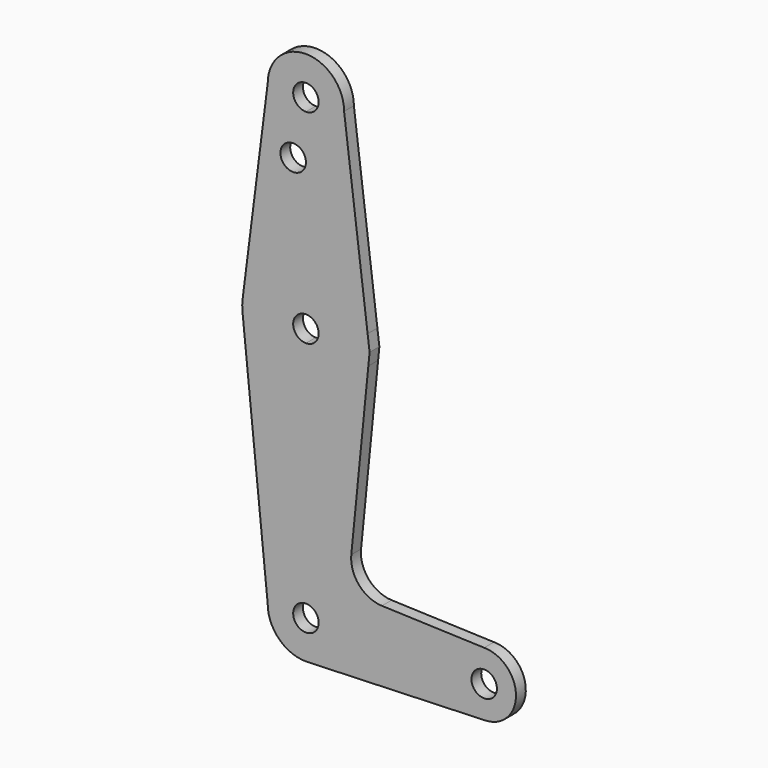
from build123d import *

# Parameters (mm, degrees)
F0_R     = 3.175
F1_DEPTH = 3.048


with BuildPart() as f1:
    # F0 (on Front) → F1 (new body)
    with BuildSketch(Plane.XZ):
        with BuildLine():
            ThreePointArc((0, 3.175), (2.2450640303, 2.2450640303), (3.175, 0))
            Line((3.175, 0), (9.525, 0))
            ThreePointArc((9.525, 0), (6.7351920908, 6.7351920908), (0, 9.525))
            Line((0, 9.525), (0, 3.175))
        make_face()
        with BuildLine():
            Line((9.525, 0), (3.175, 0))
            ThreePointArc((3.175, 0), (-2.2450640303, -2.2450640303), (0, 3.175))
            Line((0, 3.175), (0, 9.525))
            ThreePointArc((0, 9.525), (-6.7351920908, 6.7351920908), (-9.525, 0))
            ThreePointArc((-9.525, 0), (-6.7351920908, -6.7351920908), (0, -9.525))
            Line((0, -9.525), (0.6773435479, -9.500885786))
            ThreePointArc((0.6773435479, -9.500885786), (6.9705567315, -6.4912990883), (9.525, 0))
        make_face()
        with BuildLine():
            ThreePointArc((0, 9.525), (6.7351920908, 6.7351920908), (9.525, 0))
            Line((9.525, 0), (36.5125, 0))
            ThreePointArc((36.5125, 0), (38.8373399243, 5.6126600757), (44.45, 7.9375))
            Line((44.45, 7.9375), (18.9443021901, 8.8484177789))
            ThreePointArc((18.9443021901, 8.8484177789), (13.2409930554, 11.562802358), (11.3167370079, 17.5788523406))
            Line((11.3167370079, 17.5788523406), (15.5652161214, 60.3791552277))
            ThreePointArc((15.5652161214, 60.3791552277), (10.0616155323, 51.22076884), (0, 47.625))
            Line((0, 47.625), (0, 9.525))
        make_face()
        with BuildLine():
            Line((36.5125, 0), (9.525, 0))
            ThreePointArc((9.525, 0), (6.9705567315, -6.4912990883), (0.6773435479, -9.500885786))
            Line((0.6773435479, -9.500885786), (44.7324052746, -7.9324746146))
            ThreePointArc((44.7324052746, -7.9324746146), (38.9380895153, -5.7116327839), (36.5125, 0))
        make_face()
        with BuildLine():
            ThreePointArc((-9.525, 0), (-6.7351920908, 6.7351920908), (0, 9.525))
            Line((0, 9.525), (0, 47.625))
            ThreePointArc((0, 47.625), (-10.6447561055, 51.7227001204), (-15.7942028094, 61.9003804782))
            Line((-15.7942028094, 61.9003804782), (-9.525, 0))
        make_face()
        with BuildLine():
            ThreePointArc((44.45, 7.9375), (38.8373399243, 5.6126600757), (36.5125, 0))
            ThreePointArc((36.5125, 0), (38.9380895153, -5.7116327839), (44.7324052746, -7.9324746146))
            ThreePointArc((44.7324052746, -7.9324746146), (50.1616327839, -5.5119104847), (52.3875, 0))
            ThreePointArc((52.3875, 0), (50.0626600757, 5.6126600757), (44.45, 7.9375))
        make_face()
        with BuildLine():
            ThreePointArc((47.625, 0), (44.45, -3.175), (41.275, 0))
            ThreePointArc((41.275, 0), (44.45, 3.175), (47.625, 0))
        make_face(mode=Mode.SUBTRACT)
        with BuildLine():
            Line((0, 60.325), (0, 47.625))
            ThreePointArc((0, 47.625), (10.0616155323, 51.22076884), (15.5652161214, 60.3791552277))
            Line((15.5652161214, 60.3791552277), (15.875, 63.5))
            Line((15.875, 63.5), (15.3865384615, 67.4076923077))
            ThreePointArc((15.3865384615, 67.4076923077), (9.7463072395, 76.0309664508), (0, 79.375))
            Line((0, 79.375), (0, 66.675))
            ThreePointArc((0, 66.675), (2.2450640303, 65.7450640303), (3.175, 63.5))
            ThreePointArc((3.175, 63.5), (2.2450640303, 61.2549359697), (0, 60.325))
        make_face()
        with BuildLine():
            ThreePointArc((-15.7942028094, 61.9003804782), (-10.6447561055, 51.7227001204), (0, 47.625))
            Line((0, 47.625), (0, 60.325))
            ThreePointArc((0, 60.325), (-3.175, 63.5), (0, 66.675))
            Line((0, 66.675), (0, 79.375))
            ThreePointArc((0, 79.375), (-10.040231571, 75.7967221242), (-15.5542598667, 66.675))
            Line((-15.5542598667, 66.675), (-15.8547620749, 64.3013392219))
            ThreePointArc((-15.8547620749, 64.3013392219), (-15.8699525924, 63.0997129587), (-15.7942028094, 61.9003804782))
        make_face()
        with BuildLine():
            Line((-9.525, 114.3), (-15.5542598667, 66.675))
            ThreePointArc((-15.5542598667, 66.675), (-10.040231571, 75.7967221242), (0, 79.375))
            Line((0, 79.375), (0, 100.0252))
            Line((0, 100.0252), (0, 104.775))
            ThreePointArc((0, 104.775), (-6.7351920908, 107.5648079092), (-9.525, 114.3))
        make_face()
        with Locations((-3.175, 100.0252)):
            Circle(F0_R, mode=Mode.SUBTRACT)
        with BuildLine():
            ThreePointArc((0, 79.375), (9.7463072395, 76.0309664508), (15.3865384615, 67.4076923077))
            Line((15.3865384615, 67.4076923077), (9.525, 114.3))
            ThreePointArc((9.525, 114.3), (6.7351920908, 107.5648079092), (0, 104.775))
            Line((0, 104.775), (0, 100.0252))
            Line((0, 100.0252), (0, 79.375))
        make_face()
        with BuildLine():
            ThreePointArc((9.525, 114.3), (0, 123.825), (-9.525, 114.3))
            ThreePointArc((-9.525, 114.3), (-6.7351920908, 107.5648079092), (0, 104.775))
            ThreePointArc((0, 104.775), (6.7351920908, 107.5648079092), (9.525, 114.3))
        make_face()
        with BuildLine():
            ThreePointArc((3.175, 114.3), (2.2450640303, 112.0549359697), (0, 111.125))
            ThreePointArc((0, 111.125), (-2.2450640303, 116.5450640303), (3.175, 114.3))
        make_face(mode=Mode.SUBTRACT)
    extrude(amount=F1_DEPTH)


solid = f1.part
